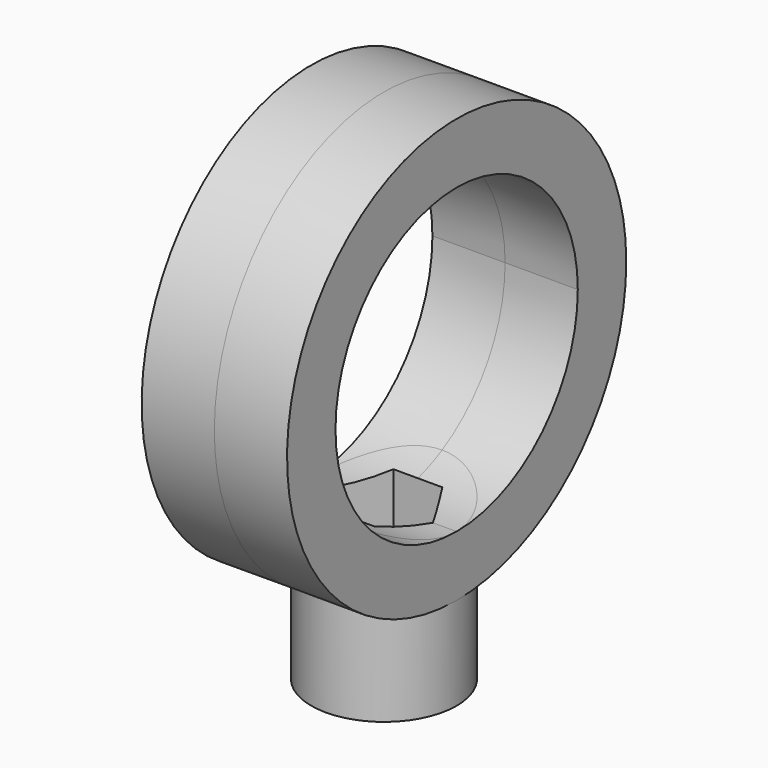
from build123d import *

# Parameters (mm, degrees)
F0_R          = 6
F0_R_2        = 2
F1_DEPTH      = 5
F2_R          = 6
F3_DEPTH      = 5
F4_R          = 17.5
F5_DEPTH      = 6
F5_DEPTH_BACK = 6
F7_END_RADIUS = 12.5
F6_R          = 6
F7_REACH      = 59.6347554857
F9_DEPTH      = 25
F10_R         = 6
F10_R_2       = 2
F11_DEPTH     = 7.5


with BuildPart() as f1:
    # F0 (on Top) → F1 (new body)
    with BuildSketch(Plane.XY):
        Circle(F0_R)
        Polygon((-4.0414518843, 0), (-2.0207259422, 3.5), (2.0207259422, 3.5), (4.0414518843, 0), (2.0207259422, -3.5), (-2.0207259422, -3.5), align=None, mode=Mode.SUBTRACT)
        Polygon((2.0207259422, 3.5), (-2.0207259422, 3.5), (-4.0414518843, 0), (-2.0207259422, -3.5), (2.0207259422, -3.5), (4.0414518843, 0), align=None)
        Circle(F0_R_2, mode=Mode.SUBTRACT)
    extrude(amount=F1_DEPTH)

    # F2 (on face) → F3 (join)
    with BuildSketch(Plane.XY.offset(5)):
        Circle(F2_R)
        Polygon((-2.5149954402, 3.1635630654), (1.482228261, 3.7598314744), (3.9972237013, 0.5962684089), (2.5149954402, -3.1635630654), (-1.482228261, -3.7598314744), (-3.9972237013, -0.5962684089), align=None, mode=Mode.SUBTRACT)
    extrude(amount=F3_DEPTH)

    # F4 (on Right) → F5 (join, two sides)
    with BuildSketch(Plane.YZ) as f5_sk:
        with Locations((0, 25.1631926373)):
            Circle(F4_R)
        with BuildLine():
            ThreePointArc((0, 12.6631926373), (-8.8388347648, 34.0020274021), (12.5, 25.1631926373))
            ThreePointArc((12.5, 25.1631926373), (8.8388347648, 16.3243578724), (0, 12.6631926373))
        make_face(mode=Mode.SUBTRACT)
    extrude(amount=-F5_DEPTH)
    extrude(f5_sk.sketch, amount=F5_DEPTH_BACK)

    f7_end = (Plane(origin=(3, 0, 25.1631926373), x_dir=(0, 0, -1), z_dir=(-1, 0, 0)) * Cylinder(F7_END_RADIUS, 232.2145957139, mode=Mode.PRIVATE)).faces().sort_by_distance((3, -12.5, 25.1631926373))[0]
    # F6 (on Top) → F7 (join, up to the whole of a round face its end follows)
    with BuildSketch(Plane.XY):
        Circle(F6_R)
    f7_long = extrude(amount=F7_REACH, mode=Mode.PRIVATE)
    add(split(f7_long, bisect_by=f7_end, keep=Keep.ALL, mode=Mode.PRIVATE).solids().sort_by_distance((0, 0, 0))[0])

    # F8 (on face) → F9 (cut)
    with BuildSketch(Plane(origin=(0, 0, 0), x_dir=(1, 0, 0), z_dir=(0, 0, -1))):
        Polygon((2.0207259422, 3.5), (-2.0207259422, 3.5), (-4.0414518843, 0), (-2.0207259422, -3.5), (2.0207259422, -3.5), (4.0414518843, 0), align=None)
    extrude(amount=-F9_DEPTH, mode=Mode.SUBTRACT)

    # F10 (on face) → F11 (join)
    with BuildSketch(Plane(origin=(0, 0, 0), x_dir=(1, 0, 0), z_dir=(0, 0, -1))):
        Circle(F10_R)
        Circle(F10_R_2, mode=Mode.SUBTRACT)
    extrude(amount=-F11_DEPTH)


solid = f1.part
